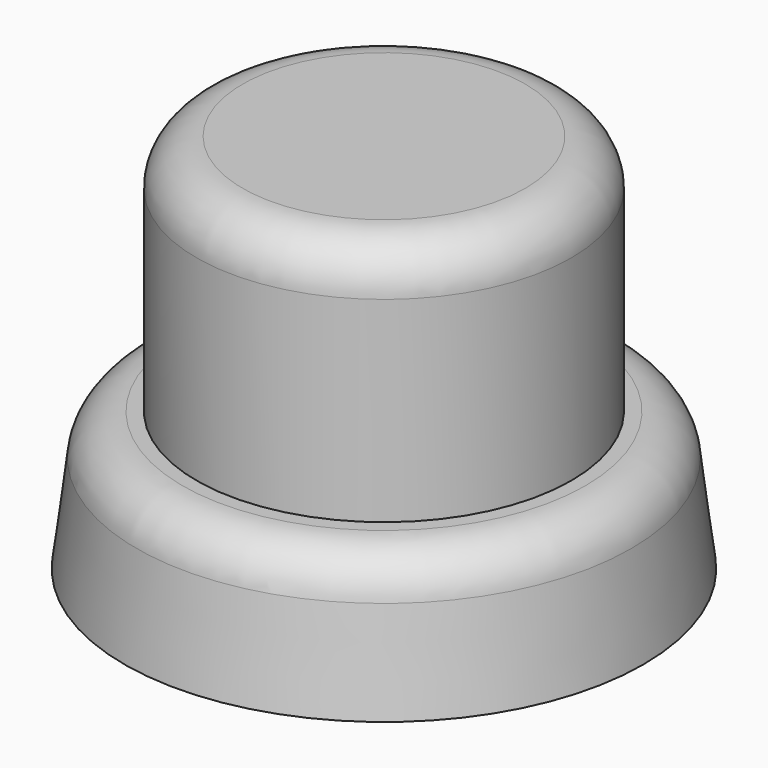
from build123d import *

# Parameters (mm, degrees)
F0_R     = 22.5
F2_R     = 21
F4_R     = 4
F5_R     = 16.25
F6_DEPTH = 21
F7_R     = 4
F8_T     = -1


with BuildPart() as f3:
    # F0 (on Top) → F3 section 0
    with BuildSketch(Plane.XY):
        Circle(F0_R)
    # F2 (on offset) → F3 section 1
    with BuildSketch(Plane.XY.offset(12)):
        Circle(F2_R)
    loft()

    # F4
    f4_edges = [f3.edges().sort_by_distance(p)[0] for p in [
        (-21, 0, 12),
    ]]
    fillet(f4_edges, radius=F4_R)

    # F5 (on face) → F6 (join)
    with BuildSketch(Plane.XY.offset(12)):
        Circle(F5_R)
    extrude(amount=F6_DEPTH)

    # F7
    f7_edges = [f3.edges().sort_by_distance(p)[0] for p in [
        (-16.25, 0, 33),
    ]]
    fillet(f7_edges, radius=F7_R)

    # F8
    f8_openings = [f3.faces().sort_by_distance(p)[0] for p in [
        (0, 0, 0),
    ]]
    offset(amount=F8_T, openings=f8_openings, kind=Kind.INTERSECTION)


solid = f3.part
